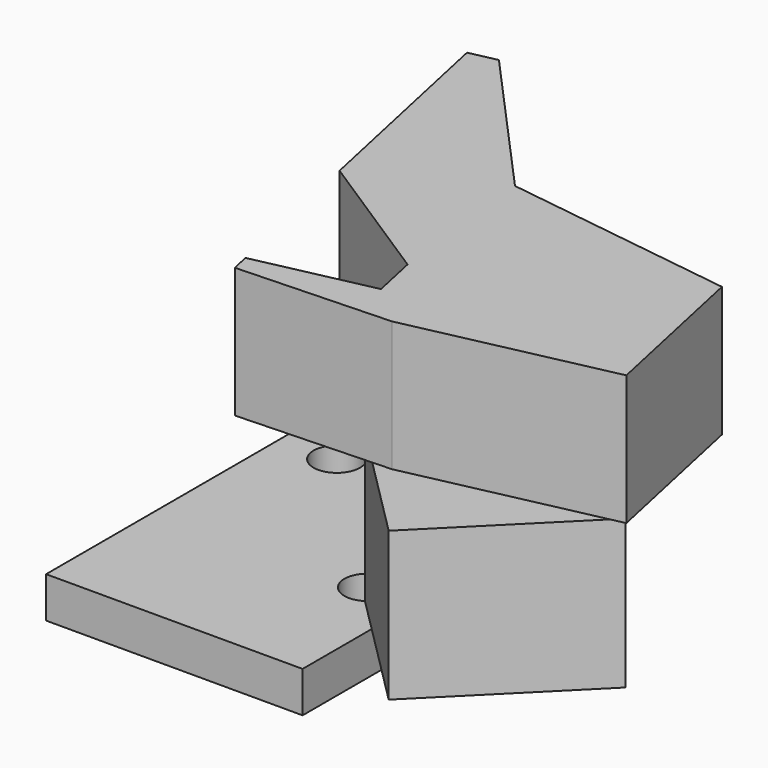
from build123d import *

# Parameters (mm, degrees)
F0_R     = 317.5
F2_DEPTH = 558.8
F4_DEPTH = 2032
F6_DEPTH = 1778


# Not quite as in the source:
# - the program builds the solid bodies; features that only make, move or delete a surface that nothing else refers to are left out


with BuildPart() as f2:
    # F0 (on Top) → F2 (new body)
    with BuildSketch(Plane.XY):
        Polygon((-2489.2, 4775.2), (-3505.2, 4775.2), (-3505.2, 4013.2), (-3505.2, 0), (0, 0), (0, 2286), (-508, 2794), align=None)
        with Locations((-2743.2, 4013.2)):
            Circle(F0_R, mode=Mode.SUBTRACT)
        with Locations((-635, 1905)):
            Circle(F0_R, mode=Mode.SUBTRACT)
    extrude(amount=-F2_DEPTH)

    # F1 (on face) → F4 (join)
    with BuildSketch(Plane.XY):
        Polygon((-3957.6947647956, 6395.1280605346), (-4316.9050096384, 6035.9178156918), (-185.9871939465, 1905), (-455.3948775786, 1635.5923163679), (1161.0512242138, 19.1462145755), (2957.1024484277, 1815.1974387893), (981.4461017924, 3790.8537854245), align=None)
    extrude(amount=F4_DEPTH)

    # F5 (on face) → F6 (join)
    with BuildSketch(Plane.XY.offset(2032)):
        Polygon((-257.708154999, 1661.5593220192), (-1837.8351896914, 1320.8298776882), (-1784.2947228834, 1072.5368684955), (300.6435319736, 1151.4881192346), (3031.8666330935, 1740.4332541235), (2550.0024318207, 3975.0703368579), (-630.3354958211, 4415.9102396305), (-2582.4618889505, 6581.5162458871), (-2954.9014027396, 6501.205545675), (-2312.4158010426, 3521.6894353624), (-391.5593220192, 2282.291845001), align=None)
    extrude(amount=F6_DEPTH)


solid = f2.part
